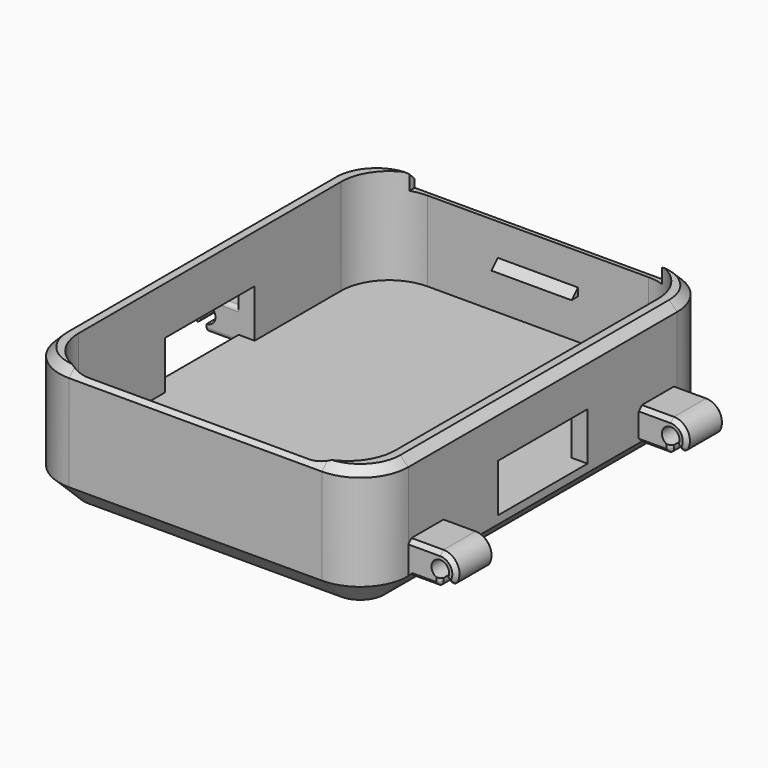
from build123d import *

# Parameters (mm, degrees)
F1_DEPTH       = 8
F3_DEPTH       = 6
F4_W           = 7
F4_H           = 3
F5_DEPTH       = 21.8
F6_W           = 15.8
F6_H           = 1
F7_DEPTH       = 3
F8_SIZE        = 1.5
F9_T1_DEPTH    = 21
F9_T3_DEPTH    = 15.8
F9_T6_ANGLE    = 114.5676286299
F9_T8_ANGLE    = 114.5676286299
F9_T10_ANGLE   = 90
F9_T12_ANGLE   = 90
F10_W          = 5
F10_H          = 2
F11_DEPTH      = 0.5
F12_T4_DEPTH   = 5
F13_W          = 3
F13_H          = 2
F14_DEPTH      = 2
F15_W          = 3
F15_H          = 1
F16_ANGLE_BACK = 113.6829972449
F16_ANGLE      = 253.6829972449
F17_W          = 3
F17_H          = 1
F18_ANGLE_BACK = 30
F18_ANGLE      = 170
F19_R          = 0.55
F20_DEPTH      = 24.0010001
F21_R          = 0.25
F22_R          = 0.25
F23_T1_DEPTH   = 1.75
F23_T3_DEPTH   = 0.842920747
F23_T8_DEPTH   = 2.392920747
F23_T13_DEPTH  = 2.392920747
F23_T16_ANGLE  = 90
F23_T18_ANGLE  = 90
F23_T20_ANGLE  = 90
F23_T22_ANGLE  = 90
F24_SIZE       = 0.24999
F25_W          = 3
F25_H          = 2
F26_DEPTH      = 2
F27_W          = 3
F27_H          = 1
F28_ANGLE_BACK = 30
F28_ANGLE      = 170
F29_W          = 3
F29_H          = 1
F30_ANGLE_BACK = 30
F30_ANGLE      = 170
F31_R          = 0.55
F32_DEPTH      = 20.0010001
F33_R          = 0.25
F34_T1_DEPTH   = 4.6910197873
F34_T3_DEPTH   = 2
F34_T5_DEPTH   = 4.25
F34_T10_DEPTH  = 2.625
F34_T15_DEPTH  = 2.625
F34_T18_ANGLE  = 175.8446845197
F34_T22_DEPTH  = 2.625
F34_T27_DEPTH  = 2.625
F34_T30_ANGLE  = 175.8446845197


# Not quite as in the source:
# - a fillet or chamfer that OpenCascade refuses, or shapes differently, is made with other operations: its cross-section is extruded or revolved along the edge and cut away or added
# - a fillet or chamfer is up to 0.001 mm smaller than in the source, because OpenCascade refuses the exact size


with BuildPart() as f1:
    # F0 (on Top) → F1 (new body)
    with BuildSketch(Plane.XY):
        with BuildLine():
            ThreePointArc((0, 3), (0.8786796564, 0.8786796564), (3, 0))
            Line((3, 0), (18.8, 0))
            ThreePointArc((18.8, 0), (20.9213203436, 0.8786796564), (21.8, 3))
            Line((21.8, 3), (21.8, 24))
            ThreePointArc((21.8, 24), (20.9213203436, 26.1213203436), (18.8, 27))
            Line((18.8, 27), (3, 27))
            ThreePointArc((3, 27), (0.8786796564, 26.1213203436), (0, 24))
            Line((0, 24), (0, 3))
        make_face()
    extrude(amount=F1_DEPTH)

    # F2 (on face) → F3 (cut)
    with BuildSketch(Plane.XY.offset(8)):
        with BuildLine():
            Line((17.8, 26.75), (4, 26.75))
            ThreePointArc((4, 26.75), (1.8786796564, 25.8713203436), (1, 23.75))
            Line((1, 23.75), (1, 3.25))
            ThreePointArc((1, 3.25), (1.8786796564, 1.1286796564), (4, 0.25))
            Line((4, 0.25), (17.8, 0.25))
            ThreePointArc((17.8, 0.25), (19.9213203436, 1.1286796564), (20.8, 3.25))
            Line((20.8, 3.25), (20.8, 23.75))
            ThreePointArc((20.8, 23.75), (19.9213203436, 25.8713203436), (17.8, 26.75))
        make_face()
    extrude(amount=-F3_DEPTH, mode=Mode.SUBTRACT)

    # F4 (on face) → F5 (cut)
    with BuildSketch(Plane.YZ.offset(21.8)):
        with Locations((13.5, 3.5)):
            Rectangle(F4_W, F4_H)
    extrude(amount=-F5_DEPTH, mode=Mode.SUBTRACT)

    # F6 (on face) → F7 (cut)
    with BuildSketch(Plane(origin=(0, 27, 0), x_dir=(-1, 0, 0), z_dir=(0, 1, 0))):
        with Locations((-10.9, 7.5)):
            Rectangle(F6_W, F6_H)
    extrude(amount=-F7_DEPTH, mode=Mode.SUBTRACT)

    # F8
    f8_edges = [f1.edges().sort_by_distance(p)[0] for p in [
        (0, 13.5, 0),
        (0.87868, 26.12132, 0),
        (0.87868, 0.87868, 0),
        (10.9, 0, 0),
        (20.92132, 0.87868, 0),
        (21.8, 13.5, 0),
        (20.92132, 26.12132, 0),
        (10.9, 27, 0),
    ]]
    chamfer(f8_edges, length=F8_SIZE)

    # F9: chamfer of 0.5 on 6 edges, made by hand

    # F9_s2 → F9_t1 (cut)
    with BuildSketch(Plane.XZ.offset(-24)):
        Polygon((0, 7.5), (0.5, 8), (0, 8), align=None)
        Polygon((21.3, 8), (21.8, 7.5), (21.8, 8), align=None)
    extrude(amount=F9_T1_DEPTH, mode=Mode.SUBTRACT)

    # F9_s4 → F9_t3 (cut)
    with BuildSketch(Plane.YZ.offset(3)):
        Polygon((0.5, 8), (0, 7.5), (0, 8), align=None)
    extrude(amount=F9_T3_DEPTH, mode=Mode.SUBTRACT)

    # F9_s5 → F9_t6 (revolve, cut)
    with BuildSketch(Plane(origin=(-6.5936613339, 3.0143088072, 0), x_dir=(0, 0, 1), z_dir=(0.9094711571, -0.4157670193, 0))):
        Polygon((7.5, -26.0746088294), (8, -25.5746088294), (8, -26.0746088294), align=None)
    revolve(axis=Axis((3, 24, 8), (0, 0, 1)), revolution_arc=F9_T6_ANGLE, mode=Mode.SUBTRACT)

    # F9_s7 → F9_t8 (revolve, cut)
    with BuildSketch(Plane.XZ.offset(-24)):
        Polygon((21.3, 8), (21.8, 7.5), (21.8, 8), align=None)
    revolve(axis=Axis((18.8, 24, 8), (0, 0, 1)), revolution_arc=F9_T8_ANGLE, mode=Mode.SUBTRACT)

    # F9_s9 → F9_t10 (revolve, cut)
    with BuildSketch(Plane.YZ.offset(18.8)):
        Polygon((0.5, 8), (0, 7.5), (0, 8), align=None)
    revolve(axis=Axis((18.8, 3, 8), (0, 0, 1)), revolution_arc=F9_T10_ANGLE, mode=Mode.SUBTRACT)

    # F9_s11 → F9_t12 (revolve, cut)
    with BuildSketch(Plane.XZ.offset(-3)):
        Polygon((0.5, 8), (0, 7.5), (0, 8), align=None)
    revolve(axis=Axis((3, 3, 8), (0, 0, 1)), revolution_arc=F9_T12_ANGLE, mode=Mode.SUBTRACT)

    # F10 (on face) → F11 (join)
    with BuildSketch(Plane.XZ.offset(-26.75)):
        with Locations((10.9, 5.5)):
            Rectangle(F10_W, F10_H)
    extrude(amount=F11_DEPTH)

    # F12: chamfer of 2 on 1 edges, made by hand


with BuildPart() as f12_tool2:
    # F12_s3 → F12_t4 (new body)
    with BuildSketch(Plane.YZ.offset(13.4)):
        Polygon((28.25, 6.5), (26.25, 4.5), (26.25, 6.5), align=None)
    extrude(amount=-F12_T4_DEPTH)

    split(bisect_by=Plane.XZ.offset(-26.75), keep=Keep.TOP)


with BuildPart() as f1_1:
    add(f1.part)

    # F12_t1: cut F12_tool2
    add(f12_tool2.part, mode=Mode.SUBTRACT)

    # F13 (on face) → F14 (join)
    with BuildSketch(Plane.YZ.offset(21.8)):
        with Locations((4.5, 2.5)):
            Rectangle(F13_W, F13_H)
        with Locations((22.5, 2.5)):
            Rectangle(F13_W, F13_H)
    extrude(amount=F14_DEPTH)

    # F15 (on face) → F16 (revolve)
    with BuildSketch(Plane.YZ.offset(23.8), mode=Mode.PRIVATE) as f16_sk:
        with Locations((4.5, 3)):
            Rectangle(F15_W, F15_H)
    revolve(f16_sk.sketch.rotate(Axis((23.8, 4.5, 2.5), (0, 1, 0)), -F16_ANGLE_BACK), axis=Axis((23.8, 4.5, 2.5), (0, 1, 0)), revolution_arc=F16_ANGLE)

    # F17 (on face) → F18 (revolve)
    with BuildSketch(Plane.YZ.offset(23.8), mode=Mode.PRIVATE) as f18_sk:
        with Locations((22.5, 3)):
            Rectangle(F17_W, F17_H)
    revolve(f18_sk.sketch.rotate(Axis((23.8, 22.5, 2.5), (0, 1, 0)), -F18_ANGLE_BACK), axis=Axis((23.8, 22.5, 2.5), (0, 1, 0)), revolution_arc=F18_ANGLE)

    # F19 (on face) → F20 (cut, through all)
    with BuildSketch(Plane(origin=(0, 24, 0), x_dir=(-1, 0, 0), z_dir=(0, 1, 0))):
        with Locations((-23.8, 2.5)):
            Circle(F19_R)
    extrude(amount=-F20_DEPTH, mode=Mode.SUBTRACT)

    # F21
    f21_edges = [f1_1.edges().sort_by_distance(p)[0] for p in [
        (23.8, 4.5, 1.5),
        (23.8, 22.5, 1.5),
    ]]
    fillet(f21_edges, radius=F21_R)

    # F22
    f22_edges = [f1_1.edges().sort_by_distance(p)[0] for p in [
        (24.442788, 4.5, 1.733956),
        (24.442788, 22.5, 1.733956),
    ]]
    fillet(f22_edges, radius=F22_R)

    # F23: chamfer of 0.25 on 4 edges, made by hand

    # F23_s2 → F23_t1 (cut)
    with BuildSketch(Plane.YZ.offset(21.8)):
        Polygon((21, 1.75), (21.25, 1.5), (21, 1.5), align=None)
        Polygon((6, 1.75), (5.75, 1.5), (6, 1.5), align=None)
    extrude(amount=F23_T1_DEPTH, mode=Mode.SUBTRACT)

    # F23_s4 → F23_t3 (cut)
    with BuildSketch(Plane.XY.offset(1.75)):
        Polygon((23.8, 23.75), (23.55, 24), (23.8, 24), align=None)
        Polygon((23.8, 3.25), (23.55, 3), (23.8, 3), align=None)
        Polygon((23.55, 6), (23.8, 5.75), (23.8, 6), align=None)
        Polygon((23.55, 21), (23.8, 21.25), (23.8, 21), align=None)
    extrude(amount=F23_T3_DEPTH, mode=Mode.SUBTRACT)


with BuildPart() as f23_tool6:
    # F23_s7 → F23_t8 (new body)
    with BuildSketch(Plane.YZ.offset(21.157079253)):
        Polygon((3.25, 1.5), (3, 1.75), (3, 1.5), align=None)
    extrude(amount=F23_T8_DEPTH)

    split(bisect_by=Plane(origin=(10.15, 0, -10.15), x_dir=(0, 1, 0), z_dir=(0.7071067812, 0, -0.7071067812)), keep=Keep.TOP)


with BuildPart() as f1_2:
    add(f1_1.part)

    # F23_t5: cut F23_tool6
    add(f23_tool6.part, mode=Mode.SUBTRACT)


with BuildPart() as f23_tool11:
    # F23_s12 → F23_t13 (new body)
    with BuildSketch(Plane.YZ.offset(21.157079253)):
        Polygon((23.75, 1.5), (24, 1.75), (24, 1.5), align=None)
    extrude(amount=F23_T13_DEPTH)

    split(bisect_by=Plane(origin=(10.15, 0, -10.15), x_dir=(0, 1, 0), z_dir=(0.7071067812, 0, -0.7071067812)), keep=Keep.TOP)


with BuildPart() as f1_3:
    add(f1_2.part)

    # F23_t10: cut F23_tool11
    add(f23_tool11.part, mode=Mode.SUBTRACT)

    # F23_s15 → F23_t16 (revolve, cut)
    with BuildSketch(Plane.XY.offset(1.75)):
        Polygon((23.8, 23.75), (23.55, 24), (23.8, 24), align=None)
    revolve(axis=Axis((23.55, 24, 1.75), (0, 1, 0)), revolution_arc=F23_T16_ANGLE, mode=Mode.SUBTRACT)

    # F23_s17 → F23_t18 (revolve, cut)
    with BuildSketch(Plane.XY.offset(1.75)):
        Polygon((23.8, 3.25), (23.55, 3), (23.8, 3), align=None)
    revolve(axis=Axis((23.55, 3, 1.75), (0, 1, 0)), revolution_arc=F23_T18_ANGLE, mode=Mode.SUBTRACT)

    # F23_s19 → F23_t20 (revolve, cut)
    with BuildSketch(Plane.XY.offset(1.75)):
        Polygon((23.55, 6), (23.8, 5.75), (23.8, 6), align=None)
    revolve(axis=Axis((23.55, 6, 1.75), (0, 1, 0)), revolution_arc=F23_T20_ANGLE, mode=Mode.SUBTRACT)

    # F23_s21 → F23_t22 (revolve, cut)
    with BuildSketch(Plane.XY.offset(1.75)):
        Polygon((23.55, 21), (23.8, 21.25), (23.8, 21), align=None)
    revolve(axis=Axis((23.55, 21, 1.75), (0, 1, 0)), revolution_arc=F23_T22_ANGLE, mode=Mode.SUBTRACT)

    # F24 (size 0.25 in the source; OpenCascade refuses exactly that, so slightly less here)
    f24_edges = [f1_3.edges().sort_by_distance(p)[0] for p in [
        (22.8, 21, 3.5),
        (24.668323, 21, 2.995998),
        (22.8, 24, 3.5),
        (22.8, 6, 3.5),
        (24.668323, 3, 2.995998),
        (22.8, 3, 3.5),
        (24.668323, 6, 2.995998),
        (24.668323, 24, 2.995998),
        (24.46667, 6, 1.869875),
        (24.204026, 6, 2.0185),
        (24.46667, 3, 1.869875),
        (24.204026, 3, 2.0185),
        (24.46667, 21, 1.869875),
        (24.204026, 21, 2.0185),
        (24.204026, 24, 2.0185),
        (24.46667, 24, 1.869875),
    ]]
    chamfer(f24_edges, length=F24_SIZE)

    # F25 (on face) → F26 (join)
    with BuildSketch(Plane(origin=(0, 0, 0), x_dir=(0, -1, 0), z_dir=(-1, 0, 0))):
        with Locations((-18.5, 2.5)):
            Rectangle(F25_W, F25_H)
        with Locations((-8.5, 2.5)):
            Rectangle(F25_W, F25_H)
    extrude(amount=F26_DEPTH)

    # F27 (on face) → F28 (revolve)
    with BuildSketch(Plane(origin=(-2, 0, 0), x_dir=(0, -1, 0), z_dir=(-1, 0, 0)), mode=Mode.PRIVATE) as f28_sk:
        with Locations((-18.5, 3)):
            Rectangle(F27_W, F27_H)
    revolve(f28_sk.sketch.rotate(Axis((-2, 18.5, 2.5), (0, -1, 0)), -F28_ANGLE_BACK), axis=Axis((-2, 18.5, 2.5), (0, -1, 0)), revolution_arc=F28_ANGLE)

    # F29 (on face) → F30 (revolve)
    with BuildSketch(Plane(origin=(-2, 0, 0), x_dir=(0, -1, 0), z_dir=(-1, 0, 0)), mode=Mode.PRIVATE) as f30_sk:
        with Locations((-8.5, 3)):
            Rectangle(F29_W, F29_H)
    revolve(f30_sk.sketch.rotate(Axis((-2, 8.5, 2.5), (0, -1, 0)), -F30_ANGLE_BACK), axis=Axis((-2, 8.5, 2.5), (0, -1, 0)), revolution_arc=F30_ANGLE)

    # F31 (on face) → F32 (cut, through all)
    with BuildSketch(Plane.XZ.offset(-7)):
        with Locations((-2, 2.5)):
            Circle(F31_R)
    extrude(amount=-F32_DEPTH, mode=Mode.SUBTRACT)

    # F33
    f33_edges = [f1_3.edges().sort_by_distance(p)[0] for p in [
        (-2.642788, 18.5, 1.733956),
        (-2.939693, 17, 2.84202),
        (-2, 18.5, 1.5),
        (-1, 20, 1.5),
        (-1, 17, 1.5),
        (-1, 20, 3.5),
        (-1, 17, 3.5),
        (-2.939693, 20, 2.84202),
    ]]
    fillet(f33_edges, radius=F33_R)

    # F34: fillet of radius 0.25 on 8 edges, made by hand

    # F34_s2 → F34_t1 (cut)
    with BuildSketch(Plane.XZ.offset(-10.8455098936)):
        with BuildLine():
            ThreePointArc((-2.8613741179, 1.9920289093), (-2.6666700685, 1.869875115), (-2.4545194777, 1.9583247796))
            Line((-2.4545194777, 1.9583247796), (-2.6427876097, 1.7339555569))
            ThreePointArc((-2.6427876097, 1.7339555569), (-2.7630701734, 1.8536843569), (-2.8613741179, 1.9920289093))
        make_face()
    extrude(amount=F34_T1_DEPTH, mode=Mode.SUBTRACT)

    # F34_s4 → F34_t3 (cut)
    with BuildSketch(Plane.YZ.offset(-2)):
        with BuildLine():
            ThreePointArc((7.25, 3.5), (7.0732233047, 3.4267766953), (7, 3.25))
            Line((7, 3.25), (7, 3.5))
            Line((7, 3.5), (7.25, 3.5))
        make_face()
        with BuildLine():
            ThreePointArc((10, 3.25), (9.9267766953, 3.4267766953), (9.75, 3.5))
            Line((9.75, 3.5), (10, 3.5))
            Line((10, 3.5), (10, 3.25))
        make_face()
    extrude(amount=F34_T3_DEPTH, mode=Mode.SUBTRACT)

    # F34_s6 → F34_t5 (cut)
    with BuildSketch(Plane.XZ.offset(-10.625)):
        with BuildLine():
            ThreePointArc((-1.75, 1.5), (-1.9267766953, 1.5732233047), (-2, 1.75))
            Line((-2, 1.75), (-2, 1.5))
            Line((-2, 1.5), (-1.75, 1.5))
        make_face()
    extrude(amount=F34_T5_DEPTH, mode=Mode.SUBTRACT)


with BuildPart() as f34_tool8:
    # F34_s9 → F34_t10 (new body)
    with BuildSketch(Plane.YZ):
        with BuildLine():
            ThreePointArc((10, 1.75), (9.9267766953, 1.5732233047), (9.75, 1.5))
            Line((9.75, 1.5), (10, 1.5))
            Line((10, 1.5), (10, 1.75))
        make_face()
    extrude(amount=-F34_T10_DEPTH)

    split(bisect_by=Plane(origin=(0.75, 0, 0.75), x_dir=(0, 1, 0), z_dir=(0.7071067812, 0, 0.7071067812)), keep=Keep.TOP)


with BuildPart() as f1_4:
    add(f1_3.part)

    # F34_t7: cut F34_tool8
    add(f34_tool8.part, mode=Mode.SUBTRACT)


with BuildPart() as f34_tool13:
    # F34_s14 → F34_t15 (new body)
    with BuildSketch(Plane.YZ):
        with BuildLine():
            ThreePointArc((10, 1.75), (9.9267766953, 1.5732233047), (9.75, 1.5))
            Line((9.75, 1.5), (10, 1.5))
            Line((10, 1.5), (10, 1.75))
        make_face()
    extrude(amount=-F34_T15_DEPTH)

    split(bisect_by=Plane(origin=(0.75, 0, 0.75), x_dir=(0, 1, 0), z_dir=(-0.7071067812, 0, -0.7071067812)), keep=Keep.TOP)


with BuildPart() as f1_5:
    add(f1_4.part)

    # F34_t12: cut F34_tool13
    add(f34_tool13.part, mode=Mode.SUBTRACT)

    # F34_s17 → F34_t18 (revolve, cut)
    with BuildSketch(Plane.YZ.offset(-2)):
        with BuildLine():
            ThreePointArc((7, 3.25), (7.0732233047, 3.4267766953), (7.25, 3.5))
            Line((7.25, 3.5), (7, 3.5))
            Line((7, 3.5), (7, 3.25))
        make_face()
    revolve(axis=Axis((-2, 7, 2.5), (0, -1, 0)), revolution_arc=F34_T18_ANGLE, mode=Mode.SUBTRACT)


with BuildPart() as f34_tool20:
    # F34_s21 → F34_t22 (new body)
    with BuildSketch(Plane.YZ):
        with BuildLine():
            ThreePointArc((7, 1.75), (7.0732233047, 1.5732233047), (7.25, 1.5))
            Line((7.25, 1.5), (7, 1.5))
            Line((7, 1.5), (7, 1.75))
        make_face()
    extrude(amount=-F34_T22_DEPTH)

    split(bisect_by=Plane(origin=(0.75, 0, 0.75), x_dir=(0, 1, 0), z_dir=(0.7071067812, 0, 0.7071067812)), keep=Keep.TOP)


with BuildPart() as f1_6:
    add(f1_5.part)

    # F34_t19: cut F34_tool20
    add(f34_tool20.part, mode=Mode.SUBTRACT)


with BuildPart() as f34_tool25:
    # F34_s26 → F34_t27 (new body)
    with BuildSketch(Plane.YZ):
        with BuildLine():
            ThreePointArc((7, 1.75), (7.0732233047, 1.5732233047), (7.25, 1.5))
            Line((7.25, 1.5), (7, 1.5))
            Line((7, 1.5), (7, 1.75))
        make_face()
    extrude(amount=-F34_T27_DEPTH)

    split(bisect_by=Plane(origin=(0.75, 0, 0.75), x_dir=(0, 1, 0), z_dir=(-0.7071067812, 0, -0.7071067812)), keep=Keep.TOP)


with BuildPart() as f1_7:
    add(f1_6.part)

    # F34_t24: cut F34_tool25
    add(f34_tool25.part, mode=Mode.SUBTRACT)

    # F34_s29 → F34_t30 (revolve, cut)
    with BuildSketch(Plane.YZ.offset(-2)):
        with BuildLine():
            ThreePointArc((10, 3.25), (9.9267766953, 3.4267766953), (9.75, 3.5))
            Line((9.75, 3.5), (10, 3.5))
            Line((10, 3.5), (10, 3.25))
        make_face()
    revolve(axis=Axis((-2, 10, 2.5), (0, -1, 0)), revolution_arc=F34_T30_ANGLE, mode=Mode.SUBTRACT)


solid = f1_7.part
